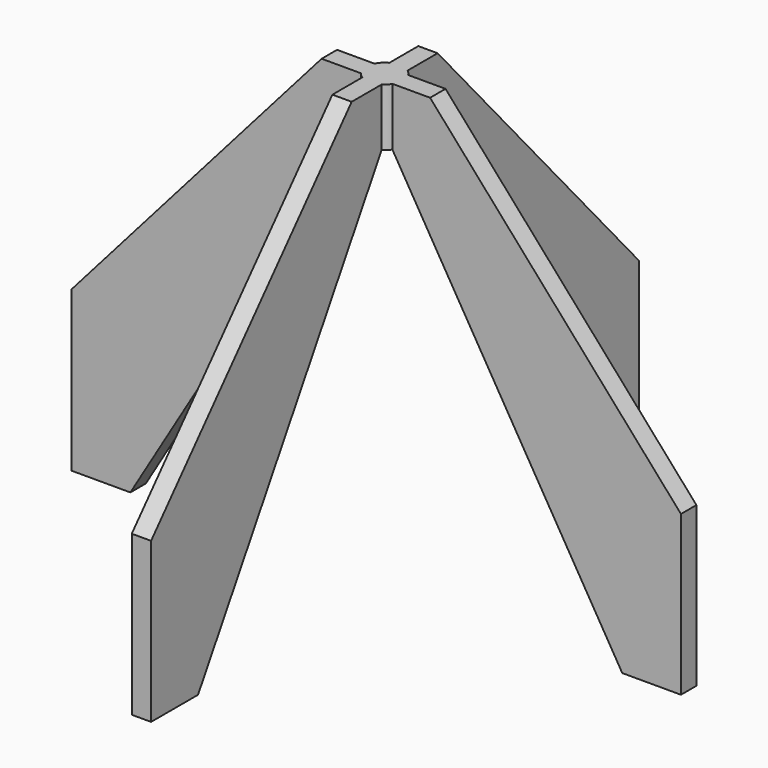
from build123d import *

# Parameters (mm, degrees)
F0_R         = 3.0488268425
F1_DEPTH     = 110
F2_W         = 3.175
F2_H         = 50
F3_DEPTH     = 80
F5_DEPTH     = 3.175
F6_W         = 50
F6_H         = 3.175
F7_DEPTH     = 80
F9_DEPTH     = 3.2191170087
F10_W        = 3.175
F10_H        = 50
F11_DEPTH    = 80
F13_DEPTH    = 3.5540803911
F14_W        = 50
F14_H        = 3.175
F15_DEPTH    = 80
F17_DEPTH    = 3.175
F18_R        = 5.3096274698
F19_DEPTH    = 5
F21_S5_R     = 3.0488268425
F21_T6_DEPTH = 9
F22_R        = 9.4311090011
F23_DEPTH    = 42
F25_DEPTH    = 3.2191170087
F27_DEPTH    = 3.6788295158
F29_DEPTH    = 3.175
F31_DEPTH    = 3.175
F32_DEPTH    = 63.5


# Not quite as in the source:
# - a fillet or chamfer that OpenCascade refuses, or shapes differently, is made with other operations: its cross-section is extruded or revolved along the edge and cut away or added


with BuildPart() as f1:
    # F0 (on Top) → F1 (new body)
    with BuildSketch(Plane.XY):
        Circle(F0_R)
    extrude(amount=F1_DEPTH)

    # F2 (on Top) → F3 (join)
    with BuildSketch(Plane.XY):
        with Locations((0.0098423844, -25)):
            Rectangle(F2_W, F2_H)
    extrude(amount=F3_DEPTH)

    # F4 (on face) → F5 (cut, through all)
    with BuildSketch(Plane(origin=(-1.5776576156, 0, 0), x_dir=(0, -1, 0), z_dir=(-1, 0, 0))):
        Polygon((50, 80), (2.6088966181, 80), (50, 26.2083634734), align=None)
    extrude(amount=-F5_DEPTH, mode=Mode.SUBTRACT)

    # F6 (on Top) → F7 (join)
    with BuildSketch(Plane.XY):
        with Locations((25, -0.0215585044)):
            Rectangle(F6_W, F6_H)
    extrude(amount=F7_DEPTH)

    # F8 (on face) → F9 (cut, through all)
    with BuildSketch(Plane.XZ.offset(1.6090585044)):
        Polygon((50, 80), (2.5896478226, 80), (50, 26.1678732932), align=None)
    extrude(amount=-F9_DEPTH, mode=Mode.SUBTRACT)

    # F10 (on Top) → F11 (join)
    with BuildSketch(Plane.XY):
        with Locations((0.1890401955, 25)):
            Rectangle(F10_W, F10_H)
    extrude(amount=F11_DEPTH)

    # F12 (on face) → F13 (cut, through all)
    with BuildSketch(Plane.YZ.offset(1.7765401955)):
        Polygon((50, 80), (2.4777510064, 80), (50, 26.2062493712), align=None)
    extrude(amount=-F13_DEPTH, mode=Mode.SUBTRACT)

    # F14 (on Top) → F15 (join)
    with BuildSketch(Plane.XY):
        with Locations((-25, -0.2514147579)):
            Rectangle(F14_W, F14_H)
    extrude(amount=F15_DEPTH)

    # F16 (on face) → F17 (cut, through all)
    with BuildSketch(Plane(origin=(0, 1.3360852421, 0), x_dir=(-1, 0, 0), z_dir=(0, 1, 0))):
        Polygon((50, 80), (2.7404783053, 80), (50, 26.2688063085), align=None)
    extrude(amount=-F17_DEPTH, mode=Mode.SUBTRACT)

    # F18 (on face) → F19 (join)
    with BuildSketch(Plane.XY.offset(110)):
        Circle(F18_R)
    extrude(amount=F19_DEPTH)

    # F21: fillet of radius 5.08 on 1 edges, made by hand


with BuildPart() as f21_tool2:
    # F21_s3 → F21_t4 (revolve)
    with BuildSketch(Plane.XZ):
        with BuildLine():
            ThreePointArc((5.3096274698, 115.08), (3.8217299183, 111.4878975516), (0.2296274698, 110))
            Line((0.2296274698, 110), (5.3096274698, 110))
            Line((5.3096274698, 110), (5.3096274698, 115.08))
        make_face()
    revolve(axis=Axis((0, 0, 110), (0, 0, 1)))

    # F21_s5 → F21_t6 (cut, symmetric)
    with BuildSketch(Plane.XY.offset(112.5)):
        Circle(F21_S5_R)
    extrude(amount=F21_T6_DEPTH, both=True, mode=Mode.SUBTRACT)


with BuildPart() as f1_1:
    add(f1.part)

    # F21_t1: cut F21_tool2
    add(f21_tool2.part, mode=Mode.SUBTRACT)

    # F22 (on face) + F20 (on face) → F23 (cut)
    with BuildSketch(Plane.XY.offset(115)):
        Circle(F22_R)
        with BuildLine():
            add(Edge.make_bspline(
                [(5.3089975095, 0), (5.3089975164, -0.1612273834), (5.3031219673, -0.3224552101), (5.2913709183, -0.483414871), (5.2737606128, -0.6438392355), (5.250323482, -0.803462652), (5.1918928197, -1.1205792461), (5.1568991277, -1.2780732959), (5.1161757966, -1.4342389448), (5.0697872067, -1.5888164279), (5.0178133896, -1.7415503683), (4.9028866804, -2.0428291895), (4.8399334722, -2.1913748989), (4.7715861919, -2.3375759551), (4.6979552247, -2.4811885599), (4.6191655532, -2.621976066), (4.4515479732, -2.8974418959), (4.3627196038, -3.0321209774), (4.2690113246, -3.163516784), (4.1705758713, -3.2914095559), (4.0675790391, -3.4155892111), (3.8528203378, -3.6561214891), (3.741057878, -3.7724747735), (3.6250912427, -3.8847148691), (3.5051104607, -3.9926533309), (3.3813166507, -4.0961135978), (3.1836352831, -4.2494509759), (3.112252337, -4.3025577734), (3.0398087405, -4.3542238063), (2.9663409133, -4.4044227305), (2.8918861372, -4.4531294369), (2.6798136644, -4.5858529875), (2.5400273484, -4.6664055795), (2.3973513324, -4.7418353748), (2.2520206742, -4.812014427), (2.1042777659, -4.876829296), (1.7114232911, -5.0323715135), (1.4627882577, -5.1142142284), (1.2095369224, -5.1812867651), (0.9527644649, -5.2332758894), (0.6935915551, -5.2699775603), (0.2946385826, -5.302637144), (0.1557563369, -5.3096254474), (0.0166889737, -5.3122478349), (-0.1223921213, -5.3104992794), (-0.2613155342, -5.3043837311), (-0.6549222008, -5.27465023), (-0.9088254061, -5.240644445), (-1.1605447695, -5.1919788406), (-1.4090280657, -5.1288359037), (-1.6532455136, -5.0514985311), (-2.0428291895, -4.9028866804), (-2.1913748989, -4.8399334722), (-2.3375759551, -4.7715861919), (-2.4811885599, -4.6979552247), (-2.621976066, -4.6191655532), (-2.9069406851, -4.4457680805), (-3.0506829028, -4.3504435211), (-3.1906552392, -4.2495537919), (-3.326590046, -4.1432865783), (-3.4582324188, -4.0318465385), (-3.7042475112, -3.8065731668), (-3.8191871972, -3.6933574313), (-3.9299611895, -3.5759895387), (-4.0363834457, -3.4546618709), (-4.1382799458, -3.3295777493), (-4.3025292517, -3.1122435833), (-4.3673403783, -3.0218507611), (-4.4298690538, -2.9298431328), (-4.4900653265, -2.8362928914), (-4.547882312, -2.7412742583), (-4.7085243801, -2.4616834099), (-4.8050260286, -2.2734759427), (-4.8924795443, -2.0807665641), (-4.9706274286, -1.8840995099), (-5.0392562783, -1.6840377697), (-5.1431777983, -1.3263374509), (-5.1825166753, -1.1698721609), (-5.2161385309, -1.0120251768), (-5.2439844367, -0.8530575539), (-5.2660114214, -0.6932334439), (-5.2955836982, -0.4000641655), (-5.304971108, -0.2669041947), (-5.3103394555, -0.1334914954), (-5.3116811185, 2.24268e-05), (-5.3089960974, 0.1334858749), (-5.2958672734, 0.3944555075), (-5.285751401, 0.5219785014), (-5.2719511359, 0.6491822874), (-5.2544795994, 0.7759339971), (-5.2333562961, 0.902101548), (-5.1784776927, 1.1802778807), (-5.1429744448, 1.3319423487), (-5.1021441975, 1.4823099163), (-5.0560473437, 1.6311473933), (-5.0047578416, 1.7782255304), (-4.893982686, 2.0632306146), (-4.8348549375, 2.2012974034), (-4.7710584997, 2.3373174414), (-4.7026828716, 2.4710941572), (-4.6298285205, 2.6024363529), (-4.5068458905, 2.8074378588), (-4.4595511931, 2.8827974536), (-4.4107459406, 2.9571984008), (-4.3604545348, 3.030602952), (-4.3087026287, 3.1029741973), (-4.1624425572, 3.2990542656), (-4.06497732, 3.4205578416), (-3.9632659712, 3.5385930737), (-3.8574636047, 3.6529756499), (-3.7477358516, 3.7635306663), (-3.5288873954, 3.9690430432), (-3.4202827483, 4.0645508664), (-3.3085859695, 4.1564837007), (-3.1939446305, 4.2447173665), (-3.0765128434, 4.3291359014), (-2.8225364614, 4.4994151645), (-2.6853493397, 4.5843188029), (-2.5451130327, 4.6641929401), (-2.4020584638, 4.7389023095), (-2.2564243419, 4.8083259132), (-1.9655922898, 4.9341801791), (-1.8205517664, 4.9909766405), (-1.6735574413, 5.0426504529), (-1.5248356135, 5.0891190703), (-1.3746170312, 5.1303133537), (-1.0662467674, 5.2033226624), (-0.9080025448, 5.2347503609), (-0.7486656211, 5.2603988366), (-0.5884996827, 5.280222352), (-0.4277707066, 5.2941912622), (-0.1057232143, 5.3103927821), (0.0555961877, 5.3126254363), (0.216942973, 5.3089765378), (0.3780495323, 5.2994488877), (0.5386489202, 5.2840615287), (0.8583007911, 5.241637974), (1.0173541533, 5.2146016616), (1.1753686742, 5.1817762024), (1.3320816823, 5.1432128436), (1.4872341021, 5.0989786844), (1.7780444639, 5.0044886665), (1.9140592952, 4.9553289334), (2.0484309855, 4.9017372808), (2.1809796225, 4.8437832023), (2.3115293435, 4.7815458821), (2.5831002543, 4.6410173426), (2.7235922798, 4.5617019911), (2.8611458759, 4.4772916377), (2.9955312596, 4.3879234765), (3.1265274005, 4.2937483988), (3.3725308355, 4.1029285715), (3.4880183137, 4.0069016419), (3.6002132702, 3.9069830353), (3.7089527961, 3.8033145651), (3.814082259, 3.6960470264), (3.9755282507, 3.5197361179), (4.0342821646, 3.4529241838), (4.0916866566, 3.3849375827), (4.1477124989, 3.3158104634), (4.2023316243, 3.2455779348), (4.594537319, 2.7197771432), (4.8754447289, 2.2216413722), (5.09088272, 1.6895647911), (5.2363259783, 1.1342583219), (5.3089977324, 0.5670131937), (5.3089975095, 0)],
                knots=[0, 0, 0, 0, 0, 0, 0, 0.0290003201, 0.0290003201, 0.0290003201, 0.0290003201, 0.0290003201, 0.0580006403, 0.0580006403, 0.0580006403, 0.0580006403, 0.0580006403, 0.0870009604, 0.0870009604, 0.0870009604, 0.0870009604, 0.0870009604, 0.1160012805, 0.1160012805, 0.1160012805, 0.1160012805, 0.1160012805, 0.1450016007, 0.1450016007, 0.1450016007, 0.1450016007, 0.1450016007, 0.1610017773, 0.1610017773, 0.1610017773, 0.1610017773, 0.1610017773, 0.1900020974, 0.1900020974, 0.1900020974, 0.1900020974, 0.1900020974, 0.2370026164, 0.2370026164, 0.2370026164, 0.2370026164, 0.2370026164, 0.2620028924, 0.2620028924, 0.2620028924, 0.2620028924, 0.2620028924, 0.3080034003, 0.3080034003, 0.3080034003, 0.3080034003, 0.3080034003, 0.3370037204, 0.3370037204, 0.3370037204, 0.3370037204, 0.3370037204, 0.3680040627, 0.3680040627, 0.3680040627, 0.3680040627, 0.3680040627, 0.3970043828, 0.3970043828, 0.3970043828, 0.3970043828, 0.3970043828, 0.4170046036, 0.4170046036, 0.4170046036, 0.4170046036, 0.4170046036, 0.4550050231, 0.4550050231, 0.4550050231, 0.4550050231, 0.4550050231, 0.4840053432, 0.4840053432, 0.4840053432, 0.4840053432, 0.4840053432, 0.5080056082, 0.5080056082, 0.5080056082, 0.5080056082, 0.5080056082, 0.5310058621, 0.5310058621, 0.5310058621, 0.5310058621, 0.5310058621, 0.5590061711, 0.5590061711, 0.5590061711, 0.5590061711, 0.5590061711, 0.5860064692, 0.5860064692, 0.5860064692, 0.5860064692, 0.5860064692, 0.6020066458, 0.6020066458, 0.6020066458, 0.6020066458, 0.6020066458, 0.6300069549, 0.6300069549, 0.6300069549, 0.6300069549, 0.6300069549, 0.6560072419, 0.6560072419, 0.6560072419, 0.6560072419, 0.6560072419, 0.6850075621, 0.6850075621, 0.6850075621, 0.6850075621, 0.6850075621, 0.7130078712, 0.7130078712, 0.7130078712, 0.7130078712, 0.7130078712, 0.7420081913, 0.7420081913, 0.7420081913, 0.7420081913, 0.7420081913, 0.7710085114, 0.7710085114, 0.7710085114, 0.7710085114, 0.7710085114, 0.8000088316, 0.8000088316, 0.8000088316, 0.8000088316, 0.8000088316, 0.8260091186, 0.8260091186, 0.8260091186, 0.8260091186, 0.8260091186, 0.8550094387, 0.8550094387, 0.8550094387, 0.8550094387, 0.8550094387, 0.8820097368, 0.8820097368, 0.8820097368, 0.8820097368, 0.8820097368, 0.8980099134, 0.8980099134, 0.8980099134, 0.8980099134, 0.8980099134, 1, 1, 1, 1, 1, 1, 1], degree=6))
        make_face(mode=Mode.SUBTRACT)
    with BuildSketch(Plane.XY.offset(115)):
        with BuildLine():
            add(Edge.make_bspline(
                [(5.3089975095, 0), (5.3089975164, -0.1612273834), (5.3031219673, -0.3224552101), (5.2913709183, -0.483414871), (5.2737606128, -0.6438392355), (5.250323482, -0.803462652), (5.1918928197, -1.1205792461), (5.1568991277, -1.2780732959), (5.1161757966, -1.4342389448), (5.0697872067, -1.5888164279), (5.0178133896, -1.7415503683), (4.9028866804, -2.0428291895), (4.8399334722, -2.1913748989), (4.7715861919, -2.3375759551), (4.6979552247, -2.4811885599), (4.6191655532, -2.621976066), (4.4515479732, -2.8974418959), (4.3627196038, -3.0321209774), (4.2690113246, -3.163516784), (4.1705758713, -3.2914095559), (4.0675790391, -3.4155892111), (3.8528203378, -3.6561214891), (3.741057878, -3.7724747735), (3.6250912427, -3.8847148691), (3.5051104607, -3.9926533309), (3.3813166507, -4.0961135978), (3.1836352831, -4.2494509759), (3.112252337, -4.3025577734), (3.0398087405, -4.3542238063), (2.9663409133, -4.4044227305), (2.8918861372, -4.4531294369), (2.6798136644, -4.5858529875), (2.5400273484, -4.6664055795), (2.3973513324, -4.7418353748), (2.2520206742, -4.812014427), (2.1042777659, -4.876829296), (1.7114232911, -5.0323715135), (1.4627882577, -5.1142142284), (1.2095369224, -5.1812867651), (0.9527644649, -5.2332758894), (0.6935915551, -5.2699775603), (0.2946385826, -5.302637144), (0.1557563369, -5.3096254474), (0.0166889737, -5.3122478349), (-0.1223921213, -5.3104992794), (-0.2613155342, -5.3043837311), (-0.6549222008, -5.27465023), (-0.9088254061, -5.240644445), (-1.1605447695, -5.1919788406), (-1.4090280657, -5.1288359037), (-1.6532455136, -5.0514985311), (-2.0428291895, -4.9028866804), (-2.1913748989, -4.8399334722), (-2.3375759551, -4.7715861919), (-2.4811885599, -4.6979552247), (-2.621976066, -4.6191655532), (-2.9069406851, -4.4457680805), (-3.0506829028, -4.3504435211), (-3.1906552392, -4.2495537919), (-3.326590046, -4.1432865783), (-3.4582324188, -4.0318465385), (-3.7042475112, -3.8065731668), (-3.8191871972, -3.6933574313), (-3.9299611895, -3.5759895387), (-4.0363834457, -3.4546618709), (-4.1382799458, -3.3295777493), (-4.3025292517, -3.1122435833), (-4.3673403783, -3.0218507611), (-4.4298690538, -2.9298431328), (-4.4900653265, -2.8362928914), (-4.547882312, -2.7412742583), (-4.7085243801, -2.4616834099), (-4.8050260286, -2.2734759427), (-4.8924795443, -2.0807665641), (-4.9706274286, -1.8840995099), (-5.0392562783, -1.6840377697), (-5.1431777983, -1.3263374509), (-5.1825166753, -1.1698721609), (-5.2161385309, -1.0120251768), (-5.2439844367, -0.8530575539), (-5.2660114214, -0.6932334439), (-5.2955836982, -0.4000641655), (-5.304971108, -0.2669041947), (-5.3103394555, -0.1334914954), (-5.3116811185, 2.24268e-05), (-5.3089960974, 0.1334858749), (-5.2958672734, 0.3944555075), (-5.285751401, 0.5219785014), (-5.2719511359, 0.6491822874), (-5.2544795994, 0.7759339971), (-5.2333562961, 0.902101548), (-5.1784776927, 1.1802778807), (-5.1429744448, 1.3319423487), (-5.1021441975, 1.4823099163), (-5.0560473437, 1.6311473933), (-5.0047578416, 1.7782255304), (-4.893982686, 2.0632306146), (-4.8348549375, 2.2012974034), (-4.7710584997, 2.3373174414), (-4.7026828716, 2.4710941572), (-4.6298285205, 2.6024363529), (-4.5068458905, 2.8074378588), (-4.4595511931, 2.8827974536), (-4.4107459406, 2.9571984008), (-4.3604545348, 3.030602952), (-4.3087026287, 3.1029741973), (-4.1624425572, 3.2990542656), (-4.06497732, 3.4205578416), (-3.9632659712, 3.5385930737), (-3.8574636047, 3.6529756499), (-3.7477358516, 3.7635306663), (-3.5288873954, 3.9690430432), (-3.4202827483, 4.0645508664), (-3.3085859695, 4.1564837007), (-3.1939446305, 4.2447173665), (-3.0765128434, 4.3291359014), (-2.8225364614, 4.4994151645), (-2.6853493397, 4.5843188029), (-2.5451130327, 4.6641929401), (-2.4020584638, 4.7389023095), (-2.2564243419, 4.8083259132), (-1.9655922898, 4.9341801791), (-1.8205517664, 4.9909766405), (-1.6735574413, 5.0426504529), (-1.5248356135, 5.0891190703), (-1.3746170312, 5.1303133537), (-1.0662467674, 5.2033226624), (-0.9080025448, 5.2347503609), (-0.7486656211, 5.2603988366), (-0.5884996827, 5.280222352), (-0.4277707066, 5.2941912622), (-0.1057232143, 5.3103927821), (0.0555961877, 5.3126254363), (0.216942973, 5.3089765378), (0.3780495323, 5.2994488877), (0.5386489202, 5.2840615287), (0.8583007911, 5.241637974), (1.0173541533, 5.2146016616), (1.1753686742, 5.1817762024), (1.3320816823, 5.1432128436), (1.4872341021, 5.0989786844), (1.7780444639, 5.0044886665), (1.9140592952, 4.9553289334), (2.0484309855, 4.9017372808), (2.1809796225, 4.8437832023), (2.3115293435, 4.7815458821), (2.5831002543, 4.6410173426), (2.7235922798, 4.5617019911), (2.8611458759, 4.4772916377), (2.9955312596, 4.3879234765), (3.1265274005, 4.2937483988), (3.3725308355, 4.1029285715), (3.4880183137, 4.0069016419), (3.6002132702, 3.9069830353), (3.7089527961, 3.8033145651), (3.814082259, 3.6960470264), (3.9755282507, 3.5197361179), (4.0342821646, 3.4529241838), (4.0916866566, 3.3849375827), (4.1477124989, 3.3158104634), (4.2023316243, 3.2455779348), (4.594537319, 2.7197771432), (4.8754447289, 2.2216413722), (5.09088272, 1.6895647911), (5.2363259783, 1.1342583219), (5.3089977324, 0.5670131937), (5.3089975095, 0)],
                knots=[0, 0, 0, 0, 0, 0, 0, 0.0290003201, 0.0290003201, 0.0290003201, 0.0290003201, 0.0290003201, 0.0580006403, 0.0580006403, 0.0580006403, 0.0580006403, 0.0580006403, 0.0870009604, 0.0870009604, 0.0870009604, 0.0870009604, 0.0870009604, 0.1160012805, 0.1160012805, 0.1160012805, 0.1160012805, 0.1160012805, 0.1450016007, 0.1450016007, 0.1450016007, 0.1450016007, 0.1450016007, 0.1610017773, 0.1610017773, 0.1610017773, 0.1610017773, 0.1610017773, 0.1900020974, 0.1900020974, 0.1900020974, 0.1900020974, 0.1900020974, 0.2370026164, 0.2370026164, 0.2370026164, 0.2370026164, 0.2370026164, 0.2620028924, 0.2620028924, 0.2620028924, 0.2620028924, 0.2620028924, 0.3080034003, 0.3080034003, 0.3080034003, 0.3080034003, 0.3080034003, 0.3370037204, 0.3370037204, 0.3370037204, 0.3370037204, 0.3370037204, 0.3680040627, 0.3680040627, 0.3680040627, 0.3680040627, 0.3680040627, 0.3970043828, 0.3970043828, 0.3970043828, 0.3970043828, 0.3970043828, 0.4170046036, 0.4170046036, 0.4170046036, 0.4170046036, 0.4170046036, 0.4550050231, 0.4550050231, 0.4550050231, 0.4550050231, 0.4550050231, 0.4840053432, 0.4840053432, 0.4840053432, 0.4840053432, 0.4840053432, 0.5080056082, 0.5080056082, 0.5080056082, 0.5080056082, 0.5080056082, 0.5310058621, 0.5310058621, 0.5310058621, 0.5310058621, 0.5310058621, 0.5590061711, 0.5590061711, 0.5590061711, 0.5590061711, 0.5590061711, 0.5860064692, 0.5860064692, 0.5860064692, 0.5860064692, 0.5860064692, 0.6020066458, 0.6020066458, 0.6020066458, 0.6020066458, 0.6020066458, 0.6300069549, 0.6300069549, 0.6300069549, 0.6300069549, 0.6300069549, 0.6560072419, 0.6560072419, 0.6560072419, 0.6560072419, 0.6560072419, 0.6850075621, 0.6850075621, 0.6850075621, 0.6850075621, 0.6850075621, 0.7130078712, 0.7130078712, 0.7130078712, 0.7130078712, 0.7130078712, 0.7420081913, 0.7420081913, 0.7420081913, 0.7420081913, 0.7420081913, 0.7710085114, 0.7710085114, 0.7710085114, 0.7710085114, 0.7710085114, 0.8000088316, 0.8000088316, 0.8000088316, 0.8000088316, 0.8000088316, 0.8260091186, 0.8260091186, 0.8260091186, 0.8260091186, 0.8260091186, 0.8550094387, 0.8550094387, 0.8550094387, 0.8550094387, 0.8550094387, 0.8820097368, 0.8820097368, 0.8820097368, 0.8820097368, 0.8820097368, 0.8980099134, 0.8980099134, 0.8980099134, 0.8980099134, 0.8980099134, 1, 1, 1, 1, 1, 1, 1], degree=6))
        make_face()
    extrude(amount=-F23_DEPTH, mode=Mode.SUBTRACT)

    # F24 (on face) → F25 (cut, through all)
    with BuildSketch(Plane.XZ.offset(1.6090585044)):
        Polygon((2.5896478226, 51.2986071408), (2.5896478226, 0), (40.3535068035, 0), (2.5896478226, 63.4334683418), align=None)
    extrude(amount=-F25_DEPTH, mode=Mode.SUBTRACT)

    # F26 (on face) → F27 (cut, through all)
    with BuildSketch(Plane.XZ.offset(1.8389147579)):
        Polygon((-2.4318177623, 63.5652467608), (-40.3364486992, 0), (-2.4318177623, 0), align=None)
    extrude(amount=-F27_DEPTH, mode=Mode.SUBTRACT)

    # F28 (on face) → F29 (cut, through all)
    with BuildSketch(Plane(origin=(-1.5776576156, 0, 0), x_dir=(0, -1, 0), z_dir=(-1, 0, 0))):
        Polygon((2.6088966181, 0), (40.3542220592, 0), (2.6088966181, 63.5277628899), align=None)
    extrude(amount=-F29_DEPTH, mode=Mode.SUBTRACT)

    # F30 (on face) → F31 (cut, through all)
    with BuildSketch(Plane(origin=(-1.3984598045, 0, 0), x_dir=(0, -1, 0), z_dir=(-1, 0, 0))):
        Polygon((-2.7091798189, 63.702121377), (-40.3488315642, 0), (-2.7091798189, 0), align=None)
    extrude(amount=-F31_DEPTH, mode=Mode.SUBTRACT)

    # F32 (cut): a face of the model
    f32_faces = [f1_1.faces().sort_by_distance(p)[0] for p in [
        (0.0572129055, 0.0359617419, 0),
    ]]
    extrude(f32_faces, amount=-F32_DEPTH, mode=Mode.SUBTRACT)


solid = f1_1.part
